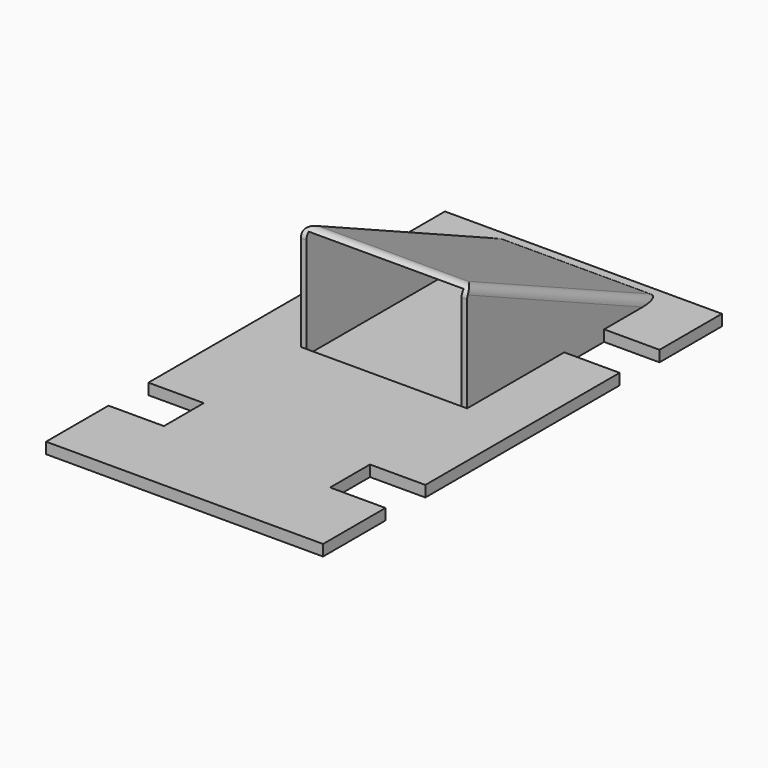
from build123d import *

# Parameters (mm, degrees)
F1_DEPTH     = 1
F3_DEPTH     = 7.5
F4_T         = 0.5
F4_T3_DEPTH  = 2
F4_T5_DEPTH  = 11.957974366
F4_T7_DEPTH  = 7.2426071697
F4_T9_DEPTH  = 16
F5_T1_DEPTH  = 21.2161866584
F5_T3_DEPTH  = 15.7001643074
F5_T8_DEPTH  = 27.8438176098
F5_T13_DEPTH = 27.8438176098


# Not quite as in the source:
# - a fillet or chamfer that OpenCascade refuses, or shapes differently, is made with other operations: its cross-section is extruded or revolved along the edge and cut away or added
# - a shell that OpenCascade refuses in one call is made with other operations: the cavity is built on its own and cut out


with BuildPart() as f1:
    # F0 (on Top) → F1 (new body)
    with BuildSketch(Plane.XY):
        Polygon((-12.5, -15.457974366), (-12.5, -22.5), (12.5, -22.5), (12.5, -15.457974366), (7.5, -15.457974366), (7.5, -10.957974366), (12.5, -10.957974366), (12.5, 10.957974366), (7.5, 10.957974366), (7.5, 15.457974366), (12.5, 15.457974366), (12.5, 22.5), (-12.5, 22.5), (-12.5, 15.457974366), (-7.5, 15.457974366), (-7.5, 10.957974366), (-12.5, 10.957974366), (-12.5, -10.957974366), (-7.5, -10.957974366), (-7.5, -15.457974366), align=None)
    extrude(amount=F1_DEPTH)

    # F2 (on Right) → F3 (join, symmetric)
    with BuildSketch(Plane.YZ):
        Polygon((21.7005815357, 0), (21.7005815357, 1.01479562), (0, 10.8946943656), (0, 0), align=None)
    extrude(amount=F3_DEPTH, both=True)

    # F4: shell of thickness 0.5, made by hand


with BuildPart() as f4_core1:
    # F4_t2: copy of F1
    add(f1.part)

    # the walls: a layer under each face that stays
    f4_faces = [f4_core1.faces().sort_by_distance(p)[0] for p in [
        (-12.5, -18.978987183, 0.5),
        (-10, -15.457974366, 0.5),
        (0, -22.5, 0.5),
        (0, 0, 0),
        (0, -5.771012817, 1),
        (-7.5, -13.207974366, 0.5),
        (12.5, -18.978987183, 0.5),
        (-10, -10.957974366, 0.5),
        (-12.5, 0, 0.5),
        (-10, 10.957974366, 0.5),
        (10, 10.957974366, 0.5),
        (12.5, 0, 0.5),
        (10, -10.957974366, 0.5),
        (7.5, -13.207974366, 0.5),
        (10, -15.457974366, 0.5),
        (-7.5, 10.8502907678, 5.4473471828),
        (7.5, 10.8502907678, 5.4473471828),
        (0, 21.7005815357, 1.00739781),
        (-8.3333333333, 16.631645305, 1),
        (0, 10.8502907678, 5.9547449928),
        (-10, 15.457974366, 0.5),
        (-12.5, 18.978987183, 0.5),
        (0, 22.5, 0.5),
        (12.5, 18.978987183, 0.5),
        (10, 15.457974366, 0.5),
    ]]
    thicken(f4_faces, amount=-F4_T, mode=Mode.SUBTRACT)

    # F4_s4 → F4_t3 (cut)
    with BuildSketch(Plane.XY.offset(-0.5)):
        Polygon((-7.505, -15.452974366), (-7.5, -15.957974366), (-7, -15.957974366), (-7, -15.457974366), align=None)
        Polygon((-7.505, -10.962974366), (-7, -10.957974366), (-7, -10.457974366), (-7.5, -10.457974366), align=None)
        Polygon((-7.505, 10.962974366), (-7.5, 10.457974366), (-7, 10.457974366), (-7, 10.957974366), align=None)
        Polygon((7.505, 10.962974366), (7.5, 10.457974366), (7, 10.457974366), (7, 10.957974366), align=None)
        Polygon((7.505, -10.962974366), (7.5, -10.457974366), (7, -10.457974366), (7, -10.957974366), align=None)
        Polygon((7.505, -15.452974366), (7, -15.457974366), (7, -15.957974366), (7.5, -15.957974366), align=None)
        Polygon((-7.505, 15.452974366), (-7, 15.457974366), (-7, 15.957974366), (-7.5, 15.957974366), align=None)
        Polygon((7.505, 15.452974366), (7, 15.457974366), (7, 15.957974366), (7.5, 15.957974366), align=None)
    extrude(amount=F4_T3_DEPTH, mode=Mode.SUBTRACT)

    # F4_s6 → F4_t5 (cut)
    with BuildSketch(Plane.XZ.offset(-11.457974366)):
        Polygon((-7.505, 1.005), (-7.5, 0.5), (-7, 0.5), (-7, 1), align=None)
        Polygon((7.505, 1.005), (7.5, 0.5), (7, 0.5), (7, 1), align=None)
    extrude(amount=F4_T5_DEPTH, mode=Mode.SUBTRACT)

    # F4_s8 → F4_t7 (cut)
    with BuildSketch(Plane.XZ.offset(-22.2005815357)):
        Polygon((-7.505, 1.005), (-7, 1), (-7, 0.5), (-7.5, 0.5), align=None)
        Polygon((7.505, 1.005), (7, 1), (7, 0.5), (7.5, 0.5), align=None)
    extrude(amount=F4_T7_DEPTH, mode=Mode.SUBTRACT)

    # F4_s10 → F4_t9 (cut)
    with BuildSketch(Plane.YZ.offset(-8)):
        Polygon((21.7055815357, 1.005), (21.2005815357, 1), (21.2005815357, 0.5), (21.7005815357, 0.5), align=None)
    extrude(amount=F4_T9_DEPTH, mode=Mode.SUBTRACT)


with BuildPart() as f1_1:
    add(f1.part)

    # what is left inside the walls is the cavity
    f4_cavity = [f4_core1.part.solids().sort_by_distance(p)[0] for p in [
        (-2.333333, 10.598219, 5.514633),
    ]]
    add(f4_cavity, mode=Mode.SUBTRACT)

    # F5: fillet of radius 0.8 on 4 edges, made by hand

    # F5_s2 → F5_t1 (cut)
    with BuildSketch(Plane.YZ.offset(-10.6080933292)):
        with BuildLine():
            ThreePointArc((0, 9.6514570339), (0.367096844, 10.3242087396), (1.1314871438, 10.3795478754))
            Line((1.1314871438, 10.3795478754), (0, 10.8946943656))
            Line((0, 10.8946943656), (0, 9.6514570339))
        make_face()
    extrude(amount=F5_T1_DEPTH, mode=Mode.SUBTRACT)

    # F5_s4 → F5_t3 (cut)
    with BuildSketch(Plane.YZ.offset(-7.8500821537)):
        with BuildLine():
            ThreePointArc((21.7005815357, 1), (21.6385322602, 1.0393388595), (21.5731357308, 1.0728194866))
            Line((21.5731357308, 1.0728194866), (21.7005815357, 1.01479562))
            Line((21.7005815357, 1.01479562), (21.7005815357, 1))
        make_face()
    extrude(amount=F5_T3_DEPTH, mode=Mode.SUBTRACT)


with BuildPart() as f5_tool6:
    # F5_s7 → F5_t8 (new body)
    with BuildSketch(Plane(origin=(0, 19.4122703842, -8.8380703302), x_dir=(1, 0, 0), z_dir=(0, -0.9101135519, 0.4143589297))):
        with BuildLine():
            ThreePointArc((-7.5, 9.1154089859), (-7.2656854249, 9.6810944108), (-6.7, 9.9154089859))
            Line((-6.7, 9.9154089859), (-7.5, 9.9154089859))
            Line((-7.5, 9.9154089859), (-7.5, 9.1154089859))
        make_face()
    extrude(amount=F5_T8_DEPTH)

    split(bisect_by=Plane.XY.offset(1), keep=Keep.TOP)


with BuildPart() as f1_2:
    add(f1_1.part)

    # F5_t5: cut F5_tool6
    add(f5_tool6.part, mode=Mode.SUBTRACT)


with BuildPart() as f5_tool11:
    # F5_s12 → F5_t13 (new body)
    with BuildSketch(Plane(origin=(0, 19.4122703842, -8.8380703302), x_dir=(1, 0, 0), z_dir=(0, -0.9101135519, 0.4143589297))):
        with BuildLine():
            ThreePointArc((7.5, 9.1154089859), (7.2656854249, 9.6810944108), (6.7, 9.9154089859))
            Line((6.7, 9.9154089859), (7.5, 9.9154089859))
            Line((7.5, 9.9154089859), (7.5, 9.1154089859))
        make_face()
    extrude(amount=F5_T13_DEPTH)

    split(bisect_by=Plane.XY.offset(1), keep=Keep.TOP)


with BuildPart() as f1_3:
    add(f1_2.part)

    # F5_t10: cut F5_tool11
    add(f5_tool11.part, mode=Mode.SUBTRACT)


solid = f1_3.part
